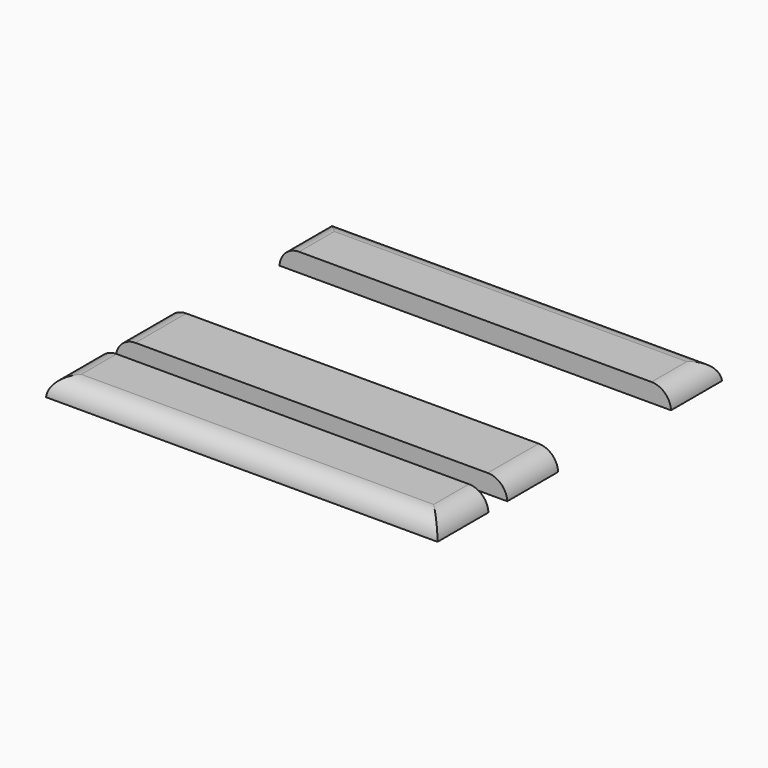
from build123d import *

# Parameters (mm, degrees)
F0_W         = 400
F0_H         = 65
F1_DEPTH     = 19
F2_W         = 400
F2_H         = 65
F3_DEPTH     = 19
F4_W         = 400
F4_H         = 65
F5_DEPTH     = 19
F6_T1_DEPTH  = 164.8749217772
F7_T1_DEPTH  = 164.8749217772
F8_T1_DEPTH  = 164.8749217772
F9_T1_DEPTH  = 479.8999374217
F10_T1_DEPTH = 144.8999374218
F11_T1_DEPTH = 164.8749217772
F12_T1_DEPTH = 479.8999374217
F13_T1_DEPTH = 144.8999374218


# Not quite as in the source:
# - a fillet or chamfer that OpenCascade refuses, or shapes differently, is made with other operations: its cross-section is extruded or revolved along the edge and cut away or added


with BuildPart() as f1:
    # F0 (on Top) → F1 (new body)
    with BuildSketch(Plane.XY):
        with Locations((-84.9136711072, 168.510709955)):
            Rectangle(F0_W, F0_H)
    extrude(amount=F1_DEPTH)

    # F6: fillet of radius 20 on 1 edges, made by hand

    # F6_s2 → F6_t1 (cut)
    with BuildSketch(Plane.XZ.offset(-250.9481708436)):
        with BuildLine():
            ThreePointArc((115.0863288928, 0), (108.8953932895, 13.4913767462), (95.1113445374, 19))
            Line((95.1113445374, 19), (115.0863288928, 19))
            Line((115.0863288928, 19), (115.0863288928, 0))
        make_face()
    extrude(amount=F6_T1_DEPTH, mode=Mode.SUBTRACT)

    # F12: fillet of radius 20 on 1 edges, made by hand

    # F12_s2 → F12_t1 (cut)
    with BuildSketch(Plane.YZ.offset(-334.8511319958)):
        with BuildLine():
            ThreePointArc((201.010709955, 0), (194.8197743517, 13.4913767462), (181.0357255996, 19))
            Line((181.0357255996, 19), (201.010709955, 19))
            Line((201.010709955, 19), (201.010709955, 0))
        make_face()
    extrude(amount=F12_T1_DEPTH, mode=Mode.SUBTRACT)

    # F13: fillet of radius 20 on 1 edges, made by hand

    # F13_s2 → F13_t1 (cut)
    with BuildSketch(Plane.XZ.offset(-230.9731864882)):
        with BuildLine():
            ThreePointArc((-284.9136711072, 0), (-278.7227355038, 13.4913767462), (-264.9386867517, 19))
            Line((-264.9386867517, 19), (-284.9136711072, 19))
            Line((-284.9136711072, 19), (-284.9136711072, 0))
        make_face()
    extrude(amount=F13_T1_DEPTH, mode=Mode.SUBTRACT)


with BuildPart() as f3:
    # F2 (on Top) → F3 (new body)
    with BuildSketch(Plane.XY):
        with Locations((-88.7223696336, -35.8872577905)):
            Rectangle(F2_W, F2_H)
    extrude(amount=F3_DEPTH)

    # F7: fillet of radius 20 on 1 edges, made by hand

    # F7_s2 → F7_t1 (cut)
    with BuildSketch(Plane.XZ.offset(-46.5502030981)):
        with BuildLine():
            ThreePointArc((111.2776303664, 0), (105.086694763, 13.4913767462), (91.3026460109, 19))
            Line((91.3026460109, 19), (111.2776303664, 19))
            Line((111.2776303664, 19), (111.2776303664, 0))
        make_face()
    extrude(amount=F7_T1_DEPTH, mode=Mode.SUBTRACT)

    # F11: fillet of radius 20 on 1 edges, made by hand

    # F11_s2 → F11_t1 (cut)
    with BuildSketch(Plane.XZ.offset(-46.5502030981)):
        with BuildLine():
            ThreePointArc((-288.7223696336, 0), (-282.5314340303, 13.4913767462), (-268.7473852782, 19))
            Line((-268.7473852782, 19), (-288.7223696336, 19))
            Line((-288.7223696336, 19), (-288.7223696336, 0))
        make_face()
    extrude(amount=F11_T1_DEPTH, mode=Mode.SUBTRACT)


with BuildPart() as f5:
    # F4 (on Top) → F5 (new body)
    with BuildSketch(Plane.XY):
        with Locations((-88.3765639737, -125.3469542844)):
            Rectangle(F4_W, F4_H)
    extrude(amount=F5_DEPTH)

    # F8: fillet of radius 20 on 1 edges, made by hand

    # F8_s2 → F8_t1 (cut)
    with BuildSketch(Plane.XZ.offset(42.9094933958)):
        with BuildLine():
            ThreePointArc((111.6234360263, 0), (105.4325004229, 13.4913767462), (91.6484516708, 19))
            Line((91.6484516708, 19), (111.6234360263, 19))
            Line((111.6234360263, 19), (111.6234360263, 0))
        make_face()
    extrude(amount=F8_T1_DEPTH, mode=Mode.SUBTRACT)

    # F9: fillet of radius 20 on 1 edges, made by hand

    # F9_s2 → F9_t1 (cut)
    with BuildSketch(Plane.YZ.offset(-338.3140248623)):
        with BuildLine():
            ThreePointArc((-137.871969929, 19), (-151.6560186811, 13.4913767462), (-157.8469542844, 0))
            Line((-157.8469542844, 0), (-157.8469542844, 19))
            Line((-157.8469542844, 19), (-137.871969929, 19))
        make_face()
    extrude(amount=F9_T1_DEPTH, mode=Mode.SUBTRACT)

    # F10: fillet of radius 20 on 1 edges, made by hand

    # F10_s2 → F10_t1 (cut)
    with BuildSketch(Plane.XZ.offset(42.9094933958)):
        with BuildLine():
            ThreePointArc((-288.3765639737, 0), (-282.1856283704, 13.4913767462), (-268.4015796183, 19))
            Line((-268.4015796183, 19), (-288.3765639737, 19))
            Line((-288.3765639737, 19), (-288.3765639737, 0))
        make_face()
    extrude(amount=F10_T1_DEPTH, mode=Mode.SUBTRACT)


solid = Compound([f1.part, f3.part, f5.part])
